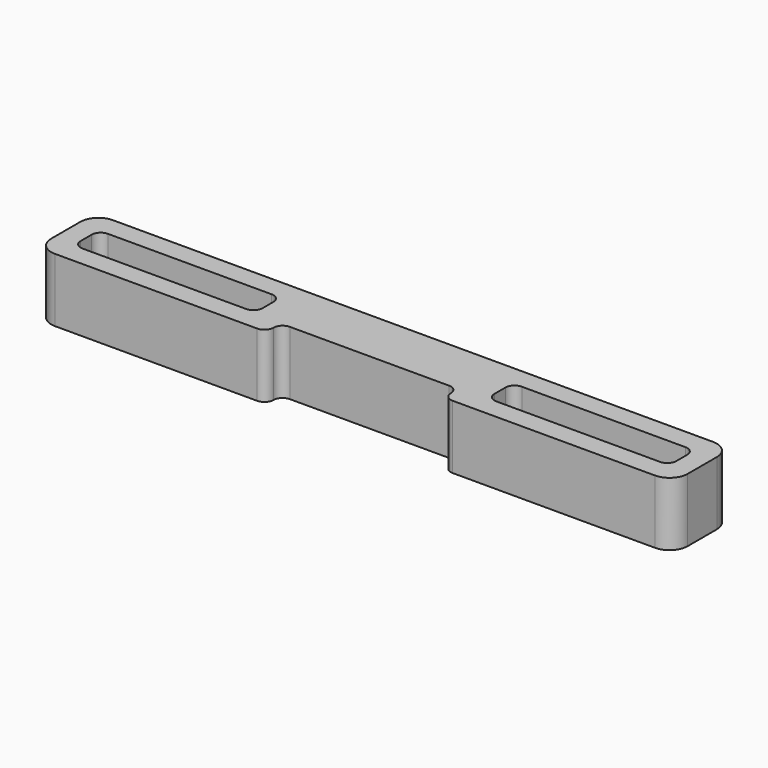
from build123d import *

# Parameters (mm, degrees)
F0_W     = 20
F0_H     = 3.5
F1_DEPTH = 7
F2_R     = 0.99999
F3_R     = 2


# Not quite as in the source:
# - two fillets or chamfers of one size are made in one step
# - a fillet or chamfer is up to 0.001 mm smaller than in the source, because OpenCascade refuses the exact size


with BuildPart() as f1:
    # F0 (on Top) → F1 (new body)
    with BuildSketch(Plane.XY):
        Polygon((35, -4), (35, 4), (-35, 4), (-35, -4), (-9.7500002012, -4), (-9.7500002012, -2), (9.75, -2), (9.75, -4), align=None)
        with Locations((-22.75, 0)):
            Rectangle(F0_W, F0_H, mode=Mode.SUBTRACT)
        with Locations((22.75, 0)):
            Rectangle(F0_W, F0_H, mode=Mode.SUBTRACT)
    extrude(amount=F1_DEPTH)

    # F2 (radius 1 in the source; OpenCascade refuses exactly that, so slightly less here)
    f2_edges = [f1.edges().sort_by_distance(p)[0] for p in [
        (32.75, 1.75, 3.5),
        (12.75, 1.75, 3.5),
        (12.75, -1.75, 3.5),
        (32.75, -1.75, 3.5),
        (-12.75, -1.75, 3.5),
        (-12.75, 1.75, 3.5),
        (-32.75, 1.75, 3.5),
        (-32.75, -1.75, 3.5),
        (-9.75, -4, 3.5),
        (-9.75, -2, 3.5),
        (9.75, -2, 3.5),
        (9.75, -4, 3.5),
    ]]
    fillet(f2_edges, radius=F2_R)

    # F3
    f3_edges = [f1.edges().sort_by_distance(p)[0] for p in [
        (35, -4, 3.5),
        (35, 4, 3.5),
        (-35, -4, 3.5),
        (-35, 4, 3.5),
    ]]
    fillet(f3_edges, radius=F3_R)


solid = f1.part
